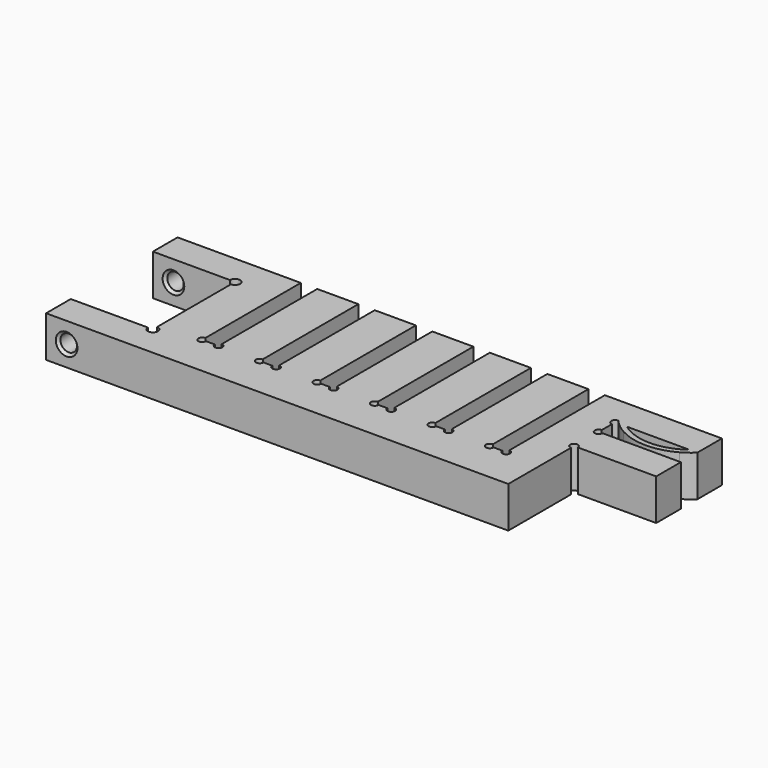
from build123d import *

# Parameters (mm, degrees)
F0_DEPTH = 12.7
F1_R     = 2.5527
F2_DEPTH = 50.801
F3_SIZE  = 0.79375
F5_DEPTH = 12.701
F6_DEPTH = 12.7
F7_W     = 25.4
F7_H     = 12.7
F8_DEPTH = 25.4
F9_DEPTH = 12.7


# Not quite as in the source:
# - a feature names something its author has since deleted; it is built from what else it names


with BuildPart() as f0:
    # F10 (on Top) → F0 (new body)
    with BuildSketch(Plane.XY):
        Polygon((-71.4375, -15.875), (-71.4375, -25.4), (71.4375, -25.4), (71.4375, 25.4), (60.6425, 25.4), (60.6425, -12.7), (55.5625, -12.7), (55.5625, 25.4), (42.8625, 25.4), (42.8625, -12.7), (37.7825, -12.7), (37.7825, 25.4), (25.0825, 25.4), (25.0825, -12.7), (20.0025, -12.7), (20.0025, 25.4), (7.3025, 25.4), (7.3025, -12.7), (2.2225, -12.7), (2.2225, 25.4), (-10.4775, 25.4), (-10.4775, -12.7), (-15.5575, -12.7), (-15.5575, 25.4), (-28.2575, 25.4), (-28.2575, -12.7), (-33.3375, -12.7), (-33.3375, 25.4), (-71.4375, 25.4), (-71.4375, 15.875), (-46.0375, 15.875), (-46.0375, -15.875), align=None)
    extrude(amount=F0_DEPTH)

    # F1 (on face) → F2 (cut, through all)
    with BuildSketch(Plane.XZ.offset(25.4)):
        with Locations((-65.0875, 6.35)):
            Circle(F1_R)
    extrude(amount=-F2_DEPTH, mode=Mode.SUBTRACT)

    # F3
    f3_edges = [f0.edges().sort_by_distance(p)[0] for p in [
        (-67.6402, 15.875, 6.35),
        (-62.5348, 20.6375, 6.35),
        (-67.6402, 25.4, 6.35),
        (-67.6402, -25.4, 6.35),
        (-62.5348, -20.6375, 6.35),
        (-67.6402, -15.875, 6.35),
    ]]
    chamfer(f3_edges, length=F3_SIZE)

    # F4 (on face) → F5 (cut, through all)
    with BuildSketch(Plane.XY.offset(12.7)):
        with BuildLine():
            ThreePointArc((-46.0375, 14.2875), (-44.9149679849, 14.7524679849), (-44.45, 15.875))
            ThreePointArc((-44.45, 15.875), (-46.0375, 17.4625), (-47.625, 15.875))
            Line((-47.625, 15.875), (-46.0375, 15.875))
            Line((-46.0375, 15.875), (-46.0375, 14.2875))
        make_face()
        with BuildLine():
            ThreePointArc((-44.45, -15.875), (-44.9149679849, -14.7524679849), (-46.0375, -14.2875))
            Line((-46.0375, -14.2875), (-46.0375, -15.875))
            Line((-46.0375, -15.875), (-47.625, -15.875))
            ThreePointArc((-47.625, -15.875), (-46.0375, -17.4625), (-44.45, -15.875))
        make_face()
    extrude(amount=-F5_DEPTH, mode=Mode.SUBTRACT)

    # F4 (on face) → F6 (cut, through all)
    with BuildSketch(Plane.XY.offset(12.7)):
        with BuildLine():
            Line((-33.3375, -12.7), (-33.3375, -11.509375))
            ThreePointArc((-33.3375, -11.509375), (-34.1793990114, -13.5418990114), (-32.146875, -12.7))
            Line((-32.146875, -12.7), (-33.3375, -12.7))
        make_face()
        with BuildLine():
            Line((-28.2575, -12.7), (-29.448125, -12.7))
            ThreePointArc((-29.448125, -12.7), (-28.2575, -13.890625), (-27.066875, -12.7))
            ThreePointArc((-27.066875, -12.7), (-27.4156009886, -11.8581009886), (-28.2575, -11.509375))
            Line((-28.2575, -11.509375), (-28.2575, -12.7))
        make_face()
        with BuildLine():
            Line((-15.5575, -12.7), (-15.5575, -11.509375))
            ThreePointArc((-15.5575, -11.509375), (-16.3993990114, -13.5418990114), (-14.366875, -12.7))
            Line((-14.366875, -12.7), (-15.5575, -12.7))
        make_face()
        with BuildLine():
            Line((-10.4775, -12.7), (-11.668125, -12.7))
            ThreePointArc((-11.668125, -12.7), (-10.4775, -13.890625), (-9.286875, -12.7))
            ThreePointArc((-9.286875, -12.7), (-9.6356009886, -11.8581009886), (-10.4775, -11.509375))
            Line((-10.4775, -11.509375), (-10.4775, -12.7))
        make_face()
        with BuildLine():
            Line((2.2225, -12.7), (2.2225, -11.509375))
            ThreePointArc((2.2225, -11.509375), (1.3806009886, -13.5418990114), (3.413125, -12.7))
            Line((3.413125, -12.7), (2.2225, -12.7))
        make_face()
        with BuildLine():
            Line((7.3025, -12.7), (6.111875, -12.7))
            ThreePointArc((6.111875, -12.7), (7.3025, -13.890625), (8.493125, -12.7))
            ThreePointArc((8.493125, -12.7), (8.1443990114, -11.8581009886), (7.3025, -11.509375))
            Line((7.3025, -11.509375), (7.3025, -12.7))
        make_face()
        with BuildLine():
            Line((20.0025, -12.7), (20.0025, -11.509375))
            ThreePointArc((20.0025, -11.509375), (19.1606009886, -13.5418990114), (21.193125, -12.7))
            Line((21.193125, -12.7), (20.0025, -12.7))
        make_face()
        with BuildLine():
            ThreePointArc((26.273125, -12.7), (25.9243990114, -11.8581009886), (25.0825, -11.509375))
            Line((25.0825, -11.509375), (25.0825, -12.7))
            Line((25.0825, -12.7), (23.891875, -12.7))
            ThreePointArc((23.891875, -12.7), (25.0825, -13.890625), (26.273125, -12.7))
        make_face()
        with BuildLine():
            ThreePointArc((37.7825, -11.509375), (36.9406009886, -13.5418990114), (38.973125, -12.7))
            Line((38.973125, -12.7), (37.7825, -12.7))
            Line((37.7825, -12.7), (37.7825, -11.509375))
        make_face()
        with BuildLine():
            ThreePointArc((44.053125, -12.7), (43.7043990114, -11.8581009886), (42.8625, -11.509375))
            Line((42.8625, -11.509375), (42.8625, -12.7))
            Line((42.8625, -12.7), (41.671875, -12.7))
            ThreePointArc((41.671875, -12.7), (42.8625, -13.890625), (44.053125, -12.7))
        make_face()
        with BuildLine():
            ThreePointArc((55.5625, -11.509375), (54.7206009886, -13.5418990114), (56.753125, -12.7))
            Line((56.753125, -12.7), (55.5625, -12.7))
            Line((55.5625, -12.7), (55.5625, -11.509375))
        make_face()
        with BuildLine():
            ThreePointArc((61.833125, -12.7), (61.4843990114, -11.8581009886), (60.6425, -11.509375))
            Line((60.6425, -11.509375), (60.6425, -12.7))
            Line((60.6425, -12.7), (59.451875, -12.7))
            ThreePointArc((59.451875, -12.7), (60.6425, -13.890625), (61.833125, -12.7))
        make_face()
    extrude(amount=-F6_DEPTH, mode=Mode.SUBTRACT)

    # F7 (on face) → F8 (join)
    with BuildSketch(Plane.YZ.offset(71.4375)):
        with Locations((12.7, 6.35)):
            Rectangle(F7_W, F7_H)
    extrude(amount=F8_DEPTH)

    # F11 (on face) → F9 (cut, through all)
    with BuildSketch(Plane.XY.offset(12.7)):
        with BuildLine():
            Line((71.4375, 10.715625), (71.4375, 9.525))
            Line((71.4375, 9.525), (72.628125, 9.525))
            ThreePointArc((72.628125, 9.525), (72.2793990114, 10.3668990114), (71.4375, 10.715625))
        make_face()
        with BuildLine():
            Line((72.628125, 9.525), (71.4375, 9.525))
            Line((71.4375, 9.525), (71.4375, 10.715625))
            ThreePointArc((71.4375, 10.715625), (70.5956009886, 8.6831009886), (72.628125, 9.525))
        make_face()
        with BuildLine():
            ThreePointArc((71.4375, 10.715625), (72.2793990114, 10.3668990114), (72.628125, 9.525))
            Line((72.628125, 9.525), (96.8375, 9.525))
            Line((96.8375, 9.525), (96.8375, 13.335))
            Line((96.8375, 13.335), (93.3474382109, 13.335))
            ThreePointArc((93.3474382109, 13.335), (84.7328125, 11.1025068978), (76.1181867891, 13.335))
            Line((76.1181867891, 13.335), (71.4375, 13.335))
            Line((71.4375, 13.335), (71.4375, 10.715625))
        make_face()
        with BuildLine():
            Line((71.4375, 14.684375), (71.4375, 13.335))
            Line((71.4375, 13.335), (76.1181867891, 13.335))
            ThreePointArc((76.1181867891, 13.335), (74.2956009479, 14.4984363954), (72.628125, 15.875))
            ThreePointArc((72.628125, 15.875), (72.2793990114, 15.0331009886), (71.4375, 14.684375))
        make_face()
        with BuildLine():
            Line((93.3474382109, 13.335), (96.8375, 13.335))
            Line((96.8375, 13.335), (96.8375, 15.875))
            ThreePointArc((96.8375, 15.875), (95.1700240521, 14.4984363954), (93.3474382109, 13.335))
        make_face()
        with BuildLine():
            ThreePointArc((71.4674857978, 17.0652473451), (70.2469694175, 15.8899940879), (71.4375, 14.684375))
            Line((71.4375, 14.684375), (71.4375, 15.875))
            Line((71.4375, 15.875), (72.628125, 15.875))
            ThreePointArc((72.628125, 15.875), (72.0338528048, 16.4565181579), (71.4674857978, 17.0652473451))
        make_face()
        with BuildLine():
            Line((71.4375, 15.875), (71.4375, 14.684375))
            ThreePointArc((71.4375, 14.684375), (72.2793990114, 15.0331009886), (72.628125, 15.875))
            Line((72.628125, 15.875), (71.4375, 15.875))
        make_face()
        with BuildLine():
            Line((71.4375, 0), (72.628125, 0))
            ThreePointArc((72.628125, 0), (70.5956009886, 0.8418990114), (71.4375, -1.190625))
            Line((71.4375, -1.190625), (71.4375, 0))
        make_face()
        with BuildLine():
            ThreePointArc((75.0951666073, 15.875), (77.5332428869, 14.378226663), (80.1971168511, 13.335))
            Line((80.1971168511, 13.335), (89.2685081489, 13.335))
            ThreePointArc((89.2685081489, 13.335), (91.9323821131, 14.378226663), (94.3704583927, 15.875))
            Line((94.3704583927, 15.875), (75.0951666073, 15.875))
        make_face()
        with BuildLine():
            Line((89.2685081489, 13.335), (80.1971168511, 13.335))
            ThreePointArc((80.1971168511, 13.335), (84.7328125, 12.6851833333), (89.2685081489, 13.335))
        make_face()
    extrude(amount=-F9_DEPTH, mode=Mode.SUBTRACT)


solid = f0.part
